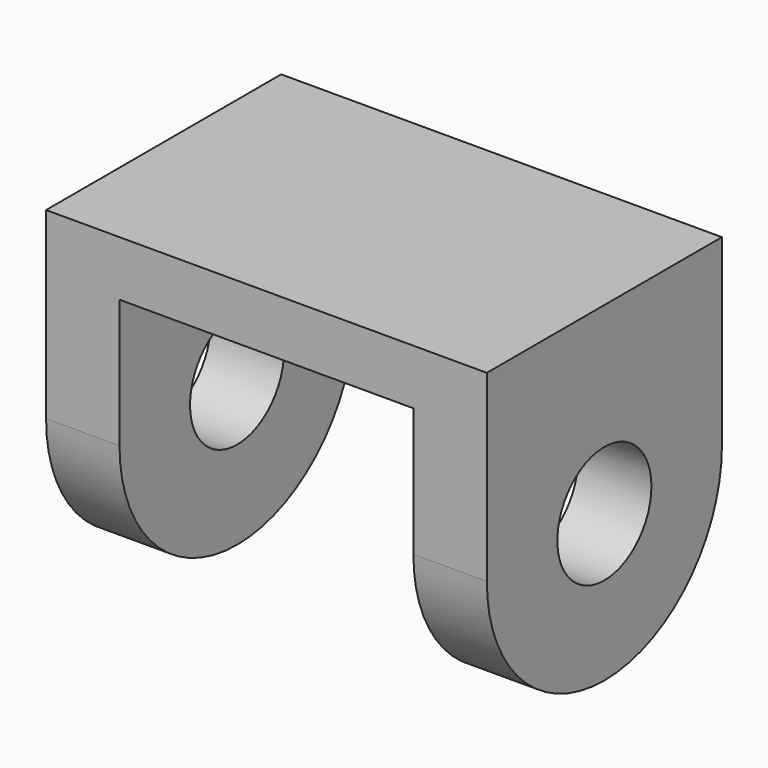
from build123d import *

# Parameters (mm, degrees)
F1_DEPTH = 80
F2_R     = 16
F3_DEPTH = 120


# Not quite as in the source:
# - the program builds the solid bodies; features that only make, move or delete a surface that nothing else refers to are left out


with BuildPart() as f1:
    # F0 (on Front) → F1 (new body)
    with BuildSketch(Plane.XZ):
        Polygon((60, -45), (60, 45), (-60, 45), (-60, -45), (-40, -45), (-40, 30), (40, 30), (40, -45), align=None)
    extrude(amount=F1_DEPTH)

    # F2 (on face) → F3 (cut)
    with BuildSketch(Plane.YZ.offset(60)):
        with BuildLine():
            ThreePointArc((-40.0000000863, -45), (-68.284271278, -33.2842712169), (-80, -5))
            Line((-80, -5), (-80, -45))
            Line((-80, -45), (-40.0000000863, -45))
        make_face()
        with BuildLine():
            Line((0, -45), (0, -5))
            ThreePointArc((0, -5), (-11.7157287831, -33.284271278), (-40.0000000863, -45))
            Line((-40.0000000863, -45), (0, -45))
        make_face()
        with Locations((-40, -5)):
            Circle(F2_R)
    extrude(amount=-F3_DEPTH, mode=Mode.SUBTRACT)


solid = f1.part
